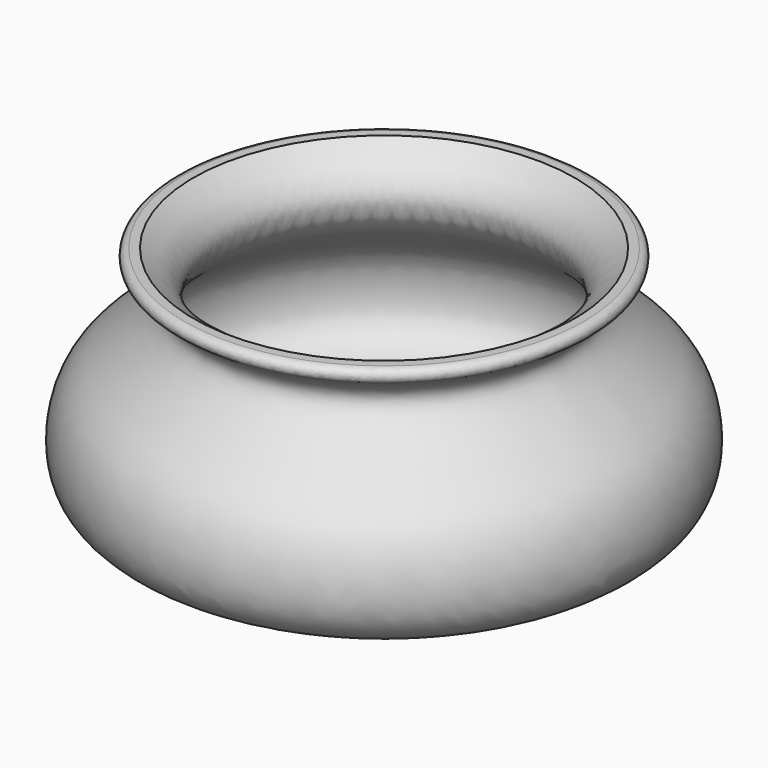
from build123d import *

# Parameters (mm, degrees)
F2_R = 1
F3_T = 2.5


# Not quite as in the source:
# - a shell that OpenCascade refuses in one call is made with other operations: the cavity is built on its own and cut out


with BuildPart() as f1:
    # F0 (on Front) → F1 (revolve)
    with BuildSketch(Plane.XZ):
        with BuildLine():
            Line((0, 36.1173562706), (0, 0))
            Line((0, 0), (20.5373205245, 0))
            add(Edge.make_bspline(
                [(32.4348025024, 36.1173562706), (28.7605769049, 34.2456221664), (21.4599230609, 30.526503016), (31.9510267097, 23.1268602371), (37.51159658, 17.9846609491), (38.2143091958, 7.603312448), (31.5622825504, 2.9212203426), (24.4903317096, 1.0474064819), (20.5373205245, 0)],
                knots=[0, 0, 0, 0, 0.1705518459, 0.338885013, 0.4979436834, 0.6622434373, 0.8112040793, 1, 1, 1, 1], degree=3))
            Line((32.4348025024, 36.1173562706), (0, 36.1173562706))
        make_face()
    revolve(axis=Axis((0, 0, 30), (0, 0, 1)))

    # F2
    f2_edges = [f1.edges().sort_by_distance(p)[0] for p in [
        (-32.434803, 0, 36.117356),
    ]]
    fillet(f2_edges, radius=F2_R)

    # F3: shell of thickness 2.5, made by hand


with BuildPart() as f3_core1:
    # F3_t2: copy of F1
    add(f1.part)

    # the walls: a layer under each face that stays
    f3_faces = [f3_core1.faces().sort_by_distance(p)[0] for p in [
        (-37.1847044397, 0, 15.5931573763),
        (-29.3924291561, 0, 35.3779908749),
        (0, 0, 0),
    ]]
    thicken(f3_faces, amount=-F3_T, mode=Mode.SUBTRACT)


with BuildPart() as f1_1:
    add(f1.part)

    # what is left inside the walls is the cavity
    f3_cavity = [f3_core1.part.solids().sort_by_distance(p)[0] for p in [
        (-31.253873, 0, 20.149337),
    ]]
    add(f3_cavity, mode=Mode.SUBTRACT)


solid = f1_1.part
